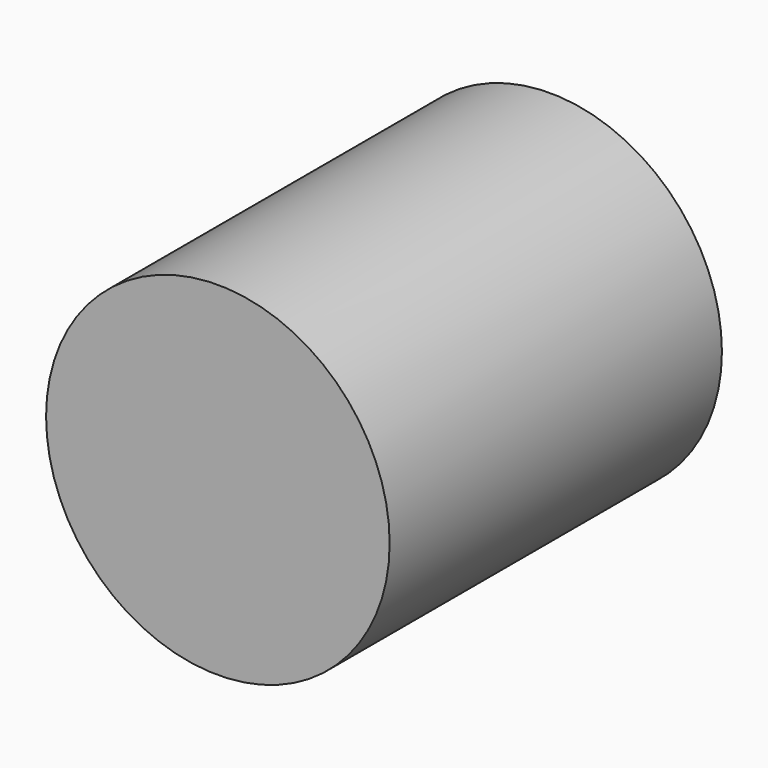
from build123d import *

# Parameters (mm, degrees)
F2_R     = 45.5060673615
F3_DEPTH = 110.0230831653


# Not quite as in the source:
# - the program builds the solid bodies; features that only make, move or delete a surface that nothing else refers to are left out


with BuildPart() as f3:
    # F2 (on Front) → F3 (new body)
    with BuildSketch(Plane.XZ):
        with Locations((-61.1175969243, 65.2746111155)):
            Circle(F2_R)
    extrude(amount=F3_DEPTH)


solid = f3.part
